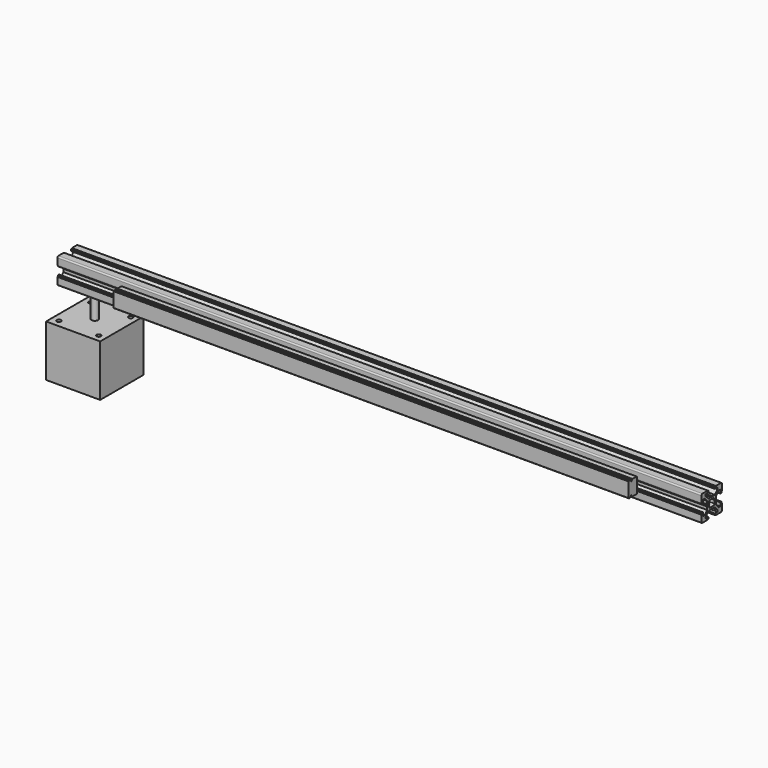
from build123d import *

# Parameters (mm, degrees)
F1_DEPTH       = 250
F1_DEPTH_BACK  = 250
F3_DEPTH       = 10
F3_DEPTH_BACK  = 10
F5_ANGLE       = 90
F7_DEPTH       = 190
F8_DEPTH       = 190
F9_W           = 42
F9_H           = 40
F10_DEPTH      = 21
F10_DEPTH_BACK = 21
F11_R          = 2.5
F12_DEPTH      = 18
F13_D          = 3.3
F13_DEPTH      = 8
F13_TIP        = 0.9914200214


with BuildPart() as f1:
    # F0 (on Right) → F1 (new body, two sides)
    with BuildSketch(Plane.YZ) as f1_sk:
        with BuildLine():
            Line((-3, 9.5), (-4, 9.5))
            Line((-4, 9.5), (-4, 10))
            Line((-4, 10), (-9, 10))
            ThreePointArc((-9, 10), (-9.7071067812, 9.7071067812), (-10, 9))
            Line((-10, 9), (-10, 4))
            Line((-10, 4), (-9.5, 4))
            Line((-9.5, 4), (-9.5, 3))
            Line((-9.5, 3), (-8.4, 3))
            Line((-8.4, 3), (-8.4, 5.8))
            Line((-8.4, 5.8), (-6.9313708499, 5.8))
            Line((-6.9313708499, 5.8), (-4.25, 3.1186291501))
            Line((-4.25, 3.1186291501), (-4.25, 0.75))
            Line((-4.25, 0.75), (-3.85, 0))
            Line((-3.85, 0), (-4.25, -0.75))
            Line((-4.25, -0.75), (-4.25, -3.1186291501))
            Line((-4.25, -3.1186291501), (-6.9313708499, -5.8))
            Line((-6.9313708499, -5.8), (-8.4, -5.8))
            Line((-8.4, -5.8), (-8.4, -3))
            Line((-8.4, -3), (-9.5, -3))
            Line((-9.5, -3), (-9.5, -4))
            Line((-9.5, -4), (-10, -4))
            Line((-10, -4), (-10, -9))
            ThreePointArc((-10, -9), (-9.7071067812, -9.7071067812), (-9, -10))
            Line((-9, -10), (-4, -10))
            Line((-4, -10), (-4, -9.5))
            Line((-4, -9.5), (-3, -9.5))
            Line((-3, -9.5), (-3, -8.4))
            Line((-3, -8.4), (-5.8, -8.4))
            Line((-5.8, -8.4), (-5.8, -6.9313708499))
            Line((-5.8, -6.9313708499), (-3.1186291501, -4.25))
            Line((-3.1186291501, -4.25), (-0.75, -4.25))
            Line((-0.75, -4.25), (0, -3.85))
            Line((0, -3.85), (0.75, -4.25))
            Line((0.75, -4.25), (3.1186291501, -4.25))
            Line((3.1186291501, -4.25), (5.8, -6.9313708499))
            Line((5.8, -6.9313708499), (5.8, -8.4))
            Line((5.8, -8.4), (3, -8.4))
            Line((3, -8.4), (3, -9.5))
            Line((3, -9.5), (4, -9.5))
            Line((4, -9.5), (4, -10))
            Line((4, -10), (9, -10))
            ThreePointArc((9, -10), (9.7071067812, -9.7071067812), (10, -9))
            Line((10, -9), (10, -4))
            Line((10, -4), (9.5, -4))
            Line((9.5, -4), (9.5, -3))
            Line((9.5, -3), (8.4, -3))
            Line((8.4, -3), (8.4, -5.8))
            Line((8.4, -5.8), (6.9313708499, -5.8))
            Line((6.9313708499, -5.8), (4.25, -3.1186291501))
            Line((4.25, -3.1186291501), (4.25, -0.75))
            Line((4.25, -0.75), (3.85, 0))
            Line((3.85, 0), (4.25, 0.75))
            Line((4.25, 0.75), (4.25, 3.1186291501))
            Line((4.25, 3.1186291501), (6.9313708499, 5.8))
            Line((6.9313708499, 5.8), (8.4, 5.8))
            Line((8.4, 5.8), (8.4, 3))
            Line((8.4, 3), (9.5, 3))
            Line((9.5, 3), (9.5, 4))
            Line((9.5, 4), (10, 4))
            Line((10, 4), (10, 9))
            ThreePointArc((10, 9), (9.7071067812, 9.7071067812), (9, 10))
            Line((9, 10), (4, 10))
            Line((4, 10), (4, 9.5))
            Line((4, 9.5), (3, 9.5))
            Line((3, 9.5), (3, 8.4))
            Line((3, 8.4), (5.8, 8.4))
            Line((5.8, 8.4), (5.8, 6.9313708499))
            Line((5.8, 6.9313708499), (3.1186291501, 4.25))
            Line((3.1186291501, 4.25), (0.75, 4.25))
            Line((0.75, 4.25), (0, 3.85))
            Line((0, 3.85), (-0.75, 4.25))
            Line((-0.75, 4.25), (-3.1186291501, 4.25))
            Line((-3.1186291501, 4.25), (-5.8, 6.9313708499))
            Line((-5.8, 6.9313708499), (-5.8, 8.4))
            Line((-5.8, 8.4), (-3, 8.4))
            Line((-3, 8.4), (-3, 9.5))
        make_face()
        with BuildLine():
            Line((1.2947580706, 2.4261289205), (1.6563032137, 2.7876740636))
            ThreePointArc((1.6563032137, 2.7876740636), (2.2926993168, 2.2926993168), (2.7876740636, 1.6563032137))
            Line((2.7876740636, 1.6563032137), (2.4261289205, 1.2947580706))
            ThreePointArc((2.4261289205, 1.2947580706), (2.75, 0), (2.4261289205, -1.2947580706))
            Line((2.4261289205, -1.2947580706), (2.7876740636, -1.6563032137))
            ThreePointArc((2.7876740636, -1.6563032137), (2.2926993168, -2.2926993168), (1.6563032137, -2.7876740636))
            Line((1.6563032137, -2.7876740636), (1.2947580706, -2.4261289205))
            ThreePointArc((1.2947580706, -2.4261289205), (0, -2.75), (-1.2947580706, -2.4261289205))
            Line((-1.2947580706, -2.4261289205), (-1.6563032137, -2.7876740636))
            ThreePointArc((-1.6563032137, -2.7876740636), (-2.2926993168, -2.2926993168), (-2.7876740636, -1.6563032137))
            Line((-2.7876740636, -1.6563032137), (-2.4261289205, -1.2947580706))
            ThreePointArc((-2.4261289205, -1.2947580706), (-2.75, 0), (-2.4261289205, 1.2947580706))
            Line((-2.4261289205, 1.2947580706), (-2.7876740636, 1.6563032137))
            ThreePointArc((-2.7876740636, 1.6563032137), (-2.2926993168, 2.2926993168), (-1.6563032137, 2.7876740636))
            Line((-1.6563032137, 2.7876740636), (-1.2947580706, 2.4261289205))
            ThreePointArc((-1.2947580706, 2.4261289205), (0, 2.75), (1.2947580706, 2.4261289205))
        make_face(mode=Mode.SUBTRACT)
    extrude(amount=F1_DEPTH)
    extrude(f1_sk.sketch, amount=-F1_DEPTH_BACK)


with BuildPart() as f3:
    # F2 (on Right) → F3 (new body, two sides)
    with BuildSketch(Plane.YZ) as f3_sk:
        with BuildLine():
            Line((5.7, 3.1613363109), (-5.7, 3.1613363109))
            Line((-5.7, 3.1613363109), (-6, 2.8613363109))
            Line((-6, 2.8613363109), (-6, 1.6111123248))
            ThreePointArc((-6, 1.6111123248), (-5.5618877209, 1.3301468843), (-5.2979118939, 0.8815928622))
            Line((-5.2979118939, 0.8815928622), (-4.687472904, 0.8815928622))
            Line((-4.687472904, 0.8815928622), (-4.687472904, 0.2435917318))
            Line((-4.687472904, 0.2435917318), (-5.2921717973, 0.2435917318))
            ThreePointArc((-5.2921717973, 0.2435917318), (-5.5549280271, -0.2169986261), (-6, -0.5052610984))
            Line((-6, -0.5052610984), (-6, -4.5386636892))
            Line((-6, -4.5386636892), (-5.7, -4.8386636892))
            Line((-5.7, -4.8386636892), (5.7, -4.8386636892))
            Line((5.7, -4.8386636892), (6, -4.5386636892))
            Line((6, -4.5386636892), (6, -0.5052610984))
            ThreePointArc((6, -0.5052610984), (5.5549280271, -0.2169986261), (5.2921717973, 0.2435917318))
            Line((5.2921717973, 0.2435917318), (4.687472904, 0.2435917318))
            Line((4.687472904, 0.2435917318), (4.687472904, 0.8815928622))
            Line((4.687472904, 0.8815928622), (5.2979118939, 0.8815928622))
            ThreePointArc((5.2979118939, 0.8815928622), (5.5618877209, 1.3301468843), (6, 1.6111123248))
            Line((6, 1.6111123248), (6, 2.8613363109))
            Line((6, 2.8613363109), (5.7, 3.1613363109))
        make_face()
    extrude(amount=F3_DEPTH)
    extrude(f3_sk.sketch, amount=-F3_DEPTH_BACK)


with BuildPart() as f3_1:
    # F5: moved
    add(f3.part.rotate(Axis((16.7408511043, 0, 0), (1, 0, 0)), F5_ANGLE))


with BuildPart() as f3_2:
    # F6: moved
    add(f3_1.part.moved(Location((0, -14.83866, 0))))

    # F7 (add): a face of the model
    f7_faces = [f3_2.faces().sort_by_distance(p)[0] for p in [
        (-10, -13.954065481, 0),
    ]]
    extrude(f7_faces, amount=F7_DEPTH)

    # F8 (add): a face of the model
    f8_faces = [f3_2.faces().sort_by_distance(p)[0] for p in [
        (10, -13.954065481, 0),
    ]]
    extrude(f8_faces, amount=F8_DEPTH)


with BuildPart() as f10:
    # F9 (on Front) → F10 (new body, two sides)
    with BuildSketch(Plane.XZ) as f10_sk:
        with Locations((-229, -50)):
            Rectangle(F9_W, F9_H)
    extrude(amount=F10_DEPTH)
    extrude(f10_sk.sketch, amount=-F10_DEPTH_BACK)

    # F11 (on face) → F12 (join)
    with BuildSketch(Plane.XY.offset(-30)):
        with Locations((-229, 0)):
            Circle(F11_R)
    extrude(amount=F12_DEPTH)

    # F13
    with Locations(Plane.XY.offset(-30)):
        with Locations((-244.5, 15.5), (-244.5, -15.5), (-213.5, -15.5), (-213.5, 15.5)):
            Hole(F13_D / 2, depth=F13_DEPTH)
            with Locations((0, 0, -(F13_DEPTH + F13_TIP / 2))):  # 118° drill point
                Cone(0, F13_D / 2, F13_TIP, mode=Mode.SUBTRACT)


solid = Compound([f1.part, f3_2.part, f10.part])
